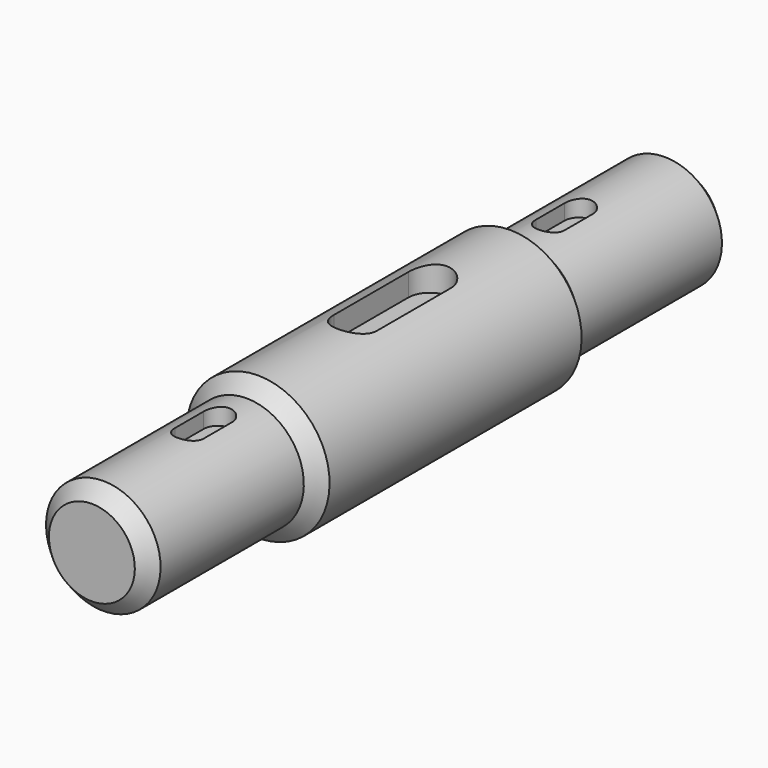
from build123d import *

# Parameters (mm, degrees)
F6_DEPTH  = 1.2
F7_SIZE   = 0.99999
F11_DEPTH = 1.8


# Not quite as in the source:
# - a fillet or chamfer is up to 0.001 mm smaller than in the source, because OpenCascade refuses the exact size
# - a pattern or mirror of a feature is missing from the dataset's text; its kind, count and spacing are read off the source's solid


with BuildPart() as f1:
    # F0 (on Right) → F1 (revolve)
    with BuildSketch(Plane.YZ):
        Polygon((0, 4), (0, 0), (51, 0), (51, 4), (37.5, 4), (37.5, 5), (13.5, 5), (13.5, 4), align=None)
    revolve(axis=Axis((0, 25.5, 0), (0, -1, 0)))

    # F5 (on offset) → F6 (cut)
    with BuildSketch(Plane.XY.offset(4)):
        with BuildLine():
            Line((1, 8.5), (1, 11))
            ThreePointArc((1, 11), (0, 12), (-1, 11))
            Line((-1, 11), (-1, 8.5))
            ThreePointArc((-1, 8.5), (0, 7.5), (1, 8.5))
        make_face()
    f6 = extrude(amount=-F6_DEPTH, mode=Mode.SUBTRACT)

    # F6_copies: F6 across plane
    add(f6.mirror(Plane(origin=(-1e-06, 25.499997, -1e-06), x_dir=(0, 0, 1), z_dir=(0, 1, 0))), mode=Mode.SUBTRACT)

    # F7 (size 1 in the source; OpenCascade refuses exactly that, so slightly less here)
    f7_edges = [f1.edges().sort_by_distance(p)[0] for p in [
        (0, 13.5, -5),
        (0, 37.5, -5),
        (0, 51, -4),
        (0, 0, -4),
    ]]
    chamfer(f7_edges, length=F7_SIZE)

    # F10 (on offset) → F11 (cut)
    with BuildSketch(Plane.XY.offset(5)):
        with BuildLine():
            Line((1.5, 23), (1.5, 29.5))
            ThreePointArc((1.5, 29.5), (0, 31), (-1.5, 29.5))
            Line((-1.5, 29.5), (-1.5, 23))
            ThreePointArc((-1.5, 23), (0, 21.5), (1.5, 23))
        make_face()
    extrude(amount=-F11_DEPTH, mode=Mode.SUBTRACT)


solid = f1.part
